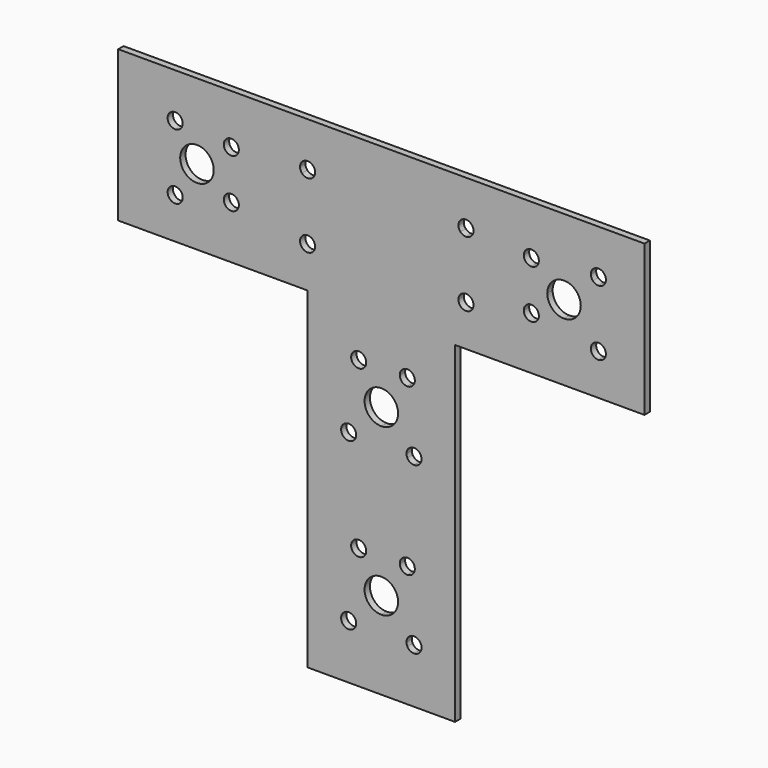
from build123d import *

# Parameters (mm, degrees)
F0_W     = 44
F0_H     = 99
F1_DEPTH = 2
F2_R     = 2.25
F2_R_2   = 5
F3_DEPTH = 2.001


with BuildPart() as f1:
    # F0 (on Front) → F1 (new body)
    with BuildSketch(Plane.XZ):
        Polygon((-78.5, 22.5), (-78.5, -22.5), (-22, -22.5), (22, -22.5), (78.5, -22.5), (78.5, 22.5), align=None)
        with Locations((0, -72)):
            Rectangle(F0_W, F0_H)
    extrude(amount=F1_DEPTH)

    # F2 (on face) → F3 (cut, through all)
    with BuildSketch(Plane.XZ.offset(2)):
        with BuildLine():
            ThreePointArc((7.75, -106.2807764064), (8.5788353904, -107.1711646096), (9.75, -107.5))
            Line((9.75, -107.5), (9.75, -105.25))
            Line((9.75, -105.25), (7.75, -105.25))
            Line((7.75, -105.25), (7.75, -106.2807764064))
        make_face()
        with BuildLine():
            Line((9.75, -105.25), (9.75, -107.5))
            ThreePointArc((9.75, -107.5), (11.3409902577, -106.8409902577), (12, -105.25))
            Line((12, -105.25), (9.75, -105.25))
        make_face()
        with BuildLine():
            Line((9.75, -103), (9.75, -105.25))
            Line((9.75, -105.25), (12, -105.25))
            ThreePointArc((12, -105.25), (11.3409902577, -103.6590097423), (9.75, -103))
        make_face()
        with BuildLine():
            Line((7.75, -105.25), (9.75, -105.25))
            Line((9.75, -105.25), (9.75, -103))
            ThreePointArc((9.75, -103), (8.5788353904, -103.3288353904), (7.75, -104.2192235936))
            Line((7.75, -104.2192235936), (7.75, -105.25))
        make_face()
        with BuildLine():
            ThreePointArc((7.5, -105.25), (7.5633930394, -105.7803300859), (7.75, -106.2807764064))
            Line((7.75, -106.2807764064), (7.75, -105.25))
            Line((7.75, -105.25), (7.5, -105.25))
        make_face()
        with Locations((-9.75, -105.25)):
            Circle(F2_R)
        with Locations((-6.75, -85.25)):
            Circle(F2_R)
        with Locations((-9.75, -55.75)):
            Circle(F2_R)
        with BuildLine():
            ThreePointArc((5, -46), (-3.5355339059, -42.4644660941), (0, -51))
            ThreePointArc((0, -51), (3.5355339059, -49.5355339059), (5, -46))
        make_face()
        with Locations((-6.75, -35.75)):
            Circle(F2_R)
        with BuildLine():
            ThreePointArc((5.5, -35.75), (6.1590097423, -37.3409902577), (7.75, -38))
            Line((7.75, -38), (7.75, -35.75))
            Line((7.75, -35.75), (5.5, -35.75))
        make_face()
        with BuildLine():
            Line((7.75, -35.75), (7.75, -38))
            ThreePointArc((7.75, -38), (9.3409902577, -37.3409902577), (10, -35.75))
            ThreePointArc((10, -35.75), (7.75, -33.5), (5.5, -35.75))
            Line((5.5, -35.75), (7.75, -35.75))
        make_face()
        with Locations((-61.5, -10.25)):
            Circle(F2_R)
        with BuildLine():
            ThreePointArc((-24.25, -10.25), (-22, -12.5), (-19.75, -10.25))
            Line((-19.75, -10.25), (-22, -10.25))
            Line((-22, -10.25), (-24.25, -10.25))
        make_face()
        with BuildLine():
            Line((-22, -10.25), (-19.75, -10.25))
            ThreePointArc((-19.75, -10.25), (-22, -8), (-24.25, -10.25))
            Line((-24.25, -10.25), (-22, -10.25))
        make_face()
        with BuildLine():
            ThreePointArc((27.5, -10.25), (26.8409902577, -8.6590097423), (25.25, -8))
            Line((25.25, -8), (25.25, -10.25))
            Line((25.25, -10.25), (23, -10.25))
            ThreePointArc((23, -10.25), (25.25, -12.5), (27.5, -10.25))
        make_face()
        with BuildLine():
            Line((25.25, -10.25), (25.25, -8))
            ThreePointArc((25.25, -8), (23.6590097423, -8.6590097423), (23, -10.25))
            Line((23, -10.25), (25.25, -10.25))
        make_face()
        with Locations((-44.75, -6.75)):
            Circle(F2_R)
        with Locations((-55, 0)):
            Circle(F2_R_2)
        with Locations((-61.5, 9.25)):
            Circle(F2_R)
        with BuildLine():
            Line((7.5, -105.25), (7.75, -105.25))
            Line((7.75, -105.25), (7.75, -104.2192235936))
            ThreePointArc((7.75, -104.2192235936), (7.5633930394, -104.7196699141), (7.5, -105.25))
        make_face()
        with BuildLine():
            ThreePointArc((0, -90.5), (-5, -95.5), (0, -100.5))
            Line((0, -100.5), (0, -95.5))
            Line((0, -95.5), (0, -90.5))
        make_face()
        with BuildLine():
            Line((0, -95.5), (0, -100.5))
            ThreePointArc((0, -100.5), (3.5355339059, -99.0355339059), (5, -95.5))
            Line((5, -95.5), (0, -95.5))
        make_face()
        with BuildLine():
            Line((9.75, -85.25), (9.75, -86.2807764064))
            ThreePointArc((9.75, -86.2807764064), (9.9366069606, -85.7803300859), (10, -85.25))
            Line((10, -85.25), (9.75, -85.25))
        make_face()
        with BuildLine():
            ThreePointArc((7.75, -87.5), (8.9211646096, -87.1711646096), (9.75, -86.2807764064))
            Line((9.75, -86.2807764064), (9.75, -85.25))
            Line((9.75, -85.25), (7.75, -85.25))
            Line((7.75, -85.25), (7.75, -87.5))
        make_face()
        with BuildLine():
            Line((0, -90.5), (0, -95.5))
            Line((0, -95.5), (5, -95.5))
            ThreePointArc((5, -95.5), (3.5355339059, -91.9644660941), (0, -90.5))
        make_face()
        with BuildLine():
            Line((9.75, -85.25), (10, -85.25))
            ThreePointArc((10, -85.25), (9.9366069606, -84.7196699141), (9.75, -84.2192235936))
            Line((9.75, -84.2192235936), (9.75, -85.25))
        make_face()
        with BuildLine():
            ThreePointArc((5.5, -85.25), (6.1590097423, -86.8409902577), (7.75, -87.5))
            Line((7.75, -87.5), (7.75, -85.25))
            Line((7.75, -85.25), (5.5, -85.25))
        make_face()
        with BuildLine():
            Line((7.75, -85.25), (9.75, -85.25))
            Line((9.75, -85.25), (9.75, -84.2192235936))
            ThreePointArc((9.75, -84.2192235936), (8.9211646096, -83.3288353904), (7.75, -83))
            Line((7.75, -83), (7.75, -85.25))
        make_face()
        with BuildLine():
            Line((5.5, -85.25), (7.75, -85.25))
            Line((7.75, -85.25), (7.75, -83))
            ThreePointArc((7.75, -83), (6.1590097423, -83.6590097423), (5.5, -85.25))
        make_face()
        with BuildLine():
            ThreePointArc((7.75, -56.7807764064), (8.5788353904, -57.6711646096), (9.75, -58))
            Line((9.75, -58), (9.75, -55.75))
            Line((9.75, -55.75), (7.75, -55.75))
            Line((7.75, -55.75), (7.75, -56.7807764064))
        make_face()
        with BuildLine():
            Line((9.75, -55.75), (9.75, -58))
            ThreePointArc((9.75, -58), (11.3409902577, -57.3409902577), (12, -55.75))
            ThreePointArc((12, -55.75), (10.2803300859, -53.5633930394), (7.75, -54.7192235936))
            Line((7.75, -54.7192235936), (7.75, -55.75))
            Line((7.75, -55.75), (9.75, -55.75))
        make_face()
        with BuildLine():
            ThreePointArc((49.5, 0), (50.9644660941, -3.5355339059), (54.5, -5))
            Line((54.5, -5), (54.5, 0))
            Line((54.5, 0), (49.5, 0))
        make_face()
        with BuildLine():
            Line((54.5, 0), (54.5, -5))
            ThreePointArc((54.5, -5), (58.0355339059, -3.5355339059), (59.5, 0))
            Line((59.5, 0), (54.5, 0))
        make_face()
        with BuildLine():
            Line((7.75, -55.75), (7.5, -55.75))
            ThreePointArc((7.5, -55.75), (7.5633930394, -56.2803300859), (7.75, -56.7807764064))
            Line((7.75, -56.7807764064), (7.75, -55.75))
        make_face()
        with BuildLine():
            ThreePointArc((7.75, -54.7192235936), (7.5633930394, -55.2196699141), (7.5, -55.75))
            Line((7.5, -55.75), (7.75, -55.75))
            Line((7.75, -55.75), (7.75, -54.7192235936))
        make_face()
        with BuildLine():
            Line((44.75, 9.25), (44.75, 10))
            ThreePointArc((44.75, 10), (43.8314413465, 9.8039595906), (43.0729490169, 9.25))
            Line((43.0729490169, 9.25), (44.75, 9.25))
        make_face()
        with BuildLine():
            ThreePointArc((46.4270509831, 9.25), (45.6685586535, 9.8039595906), (44.75, 10))
            Line((44.75, 10), (44.75, 9.25))
            Line((44.75, 9.25), (46.4270509831, 9.25))
        make_face()
        with BuildLine():
            Line((49.5, 0), (54.5, 0))
            Line((54.5, 0), (59.5, 0))
            ThreePointArc((59.5, 0), (54.5, 5), (49.5, 0))
        make_face()
        with BuildLine():
            ThreePointArc((64.75, -8), (62.5, -10.25), (64.75, -12.5))
            Line((64.75, -12.5), (64.75, -10.25))
            Line((64.75, -10.25), (64.75, -8))
        make_face()
        with BuildLine():
            Line((64.75, -10.25), (64.75, -12.5))
            ThreePointArc((64.75, -12.5), (66.3409902577, -11.8409902577), (67, -10.25))
            Line((67, -10.25), (64.75, -10.25))
        make_face()
        with BuildLine():
            ThreePointArc((47, 7.75), (46.8518878077, 8.552849702), (46.4270509831, 9.25))
            Line((46.4270509831, 9.25), (44.75, 9.25))
            Line((44.75, 9.25), (44.75, 7.75))
            Line((44.75, 7.75), (47, 7.75))
        make_face()
        with BuildLine():
            Line((44.75, 9.25), (43.0729490169, 9.25))
            ThreePointArc((43.0729490169, 9.25), (42.6481121923, 8.552849702), (42.5, 7.75))
            Line((42.5, 7.75), (44.75, 7.75))
            Line((44.75, 7.75), (44.75, 9.25))
        make_face()
        with BuildLine():
            Line((64.75, -8), (64.75, -10.25))
            Line((64.75, -10.25), (67, -10.25))
            ThreePointArc((67, -10.25), (66.3409902577, -8.6590097423), (64.75, -8))
        make_face()
        with BuildLine():
            ThreePointArc((44.75, 5.5), (46.3409902577, 6.1590097423), (47, 7.75))
            Line((47, 7.75), (44.75, 7.75))
            Line((44.75, 7.75), (44.75, 5.5))
        make_face()
        with BuildLine():
            Line((64.75, 9.25), (62.5, 9.25))
            ThreePointArc((62.5, 9.25), (62.6481121923, 8.447150298), (63.0729490169, 7.75))
            Line((63.0729490169, 7.75), (64.75, 7.75))
            Line((64.75, 7.75), (64.75, 9.25))
        make_face()
        with BuildLine():
            ThreePointArc((67, 9.25), (64.75, 11.5), (62.5, 9.25))
            Line((62.5, 9.25), (64.75, 9.25))
            Line((64.75, 9.25), (64.75, 7.75))
            Line((64.75, 7.75), (66.4270509831, 7.75))
            ThreePointArc((66.4270509831, 7.75), (66.8518878077, 8.447150298), (67, 9.25))
        make_face()
        with BuildLine():
            Line((44.75, 7.75), (42.5, 7.75))
            ThreePointArc((42.5, 7.75), (43.1590097423, 6.1590097423), (44.75, 5.5))
            Line((44.75, 5.5), (44.75, 7.75))
        make_face()
        with BuildLine():
            ThreePointArc((26.9270509831, 7.75), (27.3518878077, 8.447150298), (27.5, 9.25))
            Line((27.5, 9.25), (25.25, 9.25))
            Line((25.25, 9.25), (25.25, 7.75))
            Line((25.25, 7.75), (26.9270509831, 7.75))
        make_face()
        with BuildLine():
            Line((25.25, 9.25), (27.5, 9.25))
            ThreePointArc((27.5, 9.25), (25.25, 11.5), (23, 9.25))
            Line((23, 9.25), (25.25, 9.25))
        make_face()
        with BuildLine():
            ThreePointArc((64.75, 7), (65.6685586535, 7.1960404094), (66.4270509831, 7.75))
            Line((66.4270509831, 7.75), (64.75, 7.75))
            Line((64.75, 7.75), (64.75, 7))
        make_face()
        with BuildLine():
            ThreePointArc((47, -6.75), (46.3409902577, -5.1590097423), (44.75, -4.5))
            Line((44.75, -4.5), (44.75, -6.75))
            Line((44.75, -6.75), (42.5, -6.75))
            ThreePointArc((42.5, -6.75), (44.75, -9), (47, -6.75))
        make_face()
        with BuildLine():
            Line((44.75, -6.75), (44.75, -4.5))
            ThreePointArc((44.75, -4.5), (43.1590097423, -5.1590097423), (42.5, -6.75))
            Line((42.5, -6.75), (44.75, -6.75))
        make_face()
        with BuildLine():
            ThreePointArc((63.0729490169, 7.75), (63.8314413465, 7.1960404094), (64.75, 7))
            Line((64.75, 7), (64.75, 7.75))
            Line((64.75, 7.75), (63.0729490169, 7.75))
        make_face()
        with BuildLine():
            ThreePointArc((25.25, 7), (26.1685586535, 7.1960404094), (26.9270509831, 7.75))
            Line((26.9270509831, 7.75), (25.25, 7.75))
            Line((25.25, 7.75), (25.25, 7))
        make_face()
        with BuildLine():
            Line((25.25, 7.75), (25.25, 9.25))
            Line((25.25, 9.25), (23, 9.25))
            ThreePointArc((23, 9.25), (23.1481121923, 8.447150298), (23.5729490169, 7.75))
            Line((23.5729490169, 7.75), (25.25, 7.75))
        make_face()
        with BuildLine():
            ThreePointArc((23.5729490169, 7.75), (24.3314413465, 7.1960404094), (25.25, 7))
            Line((25.25, 7), (25.25, 7.75))
            Line((25.25, 7.75), (23.5729490169, 7.75))
        make_face()
        with BuildLine():
            ThreePointArc((-20.3229490169, 7.75), (-19.8981121923, 8.447150298), (-19.75, 9.25))
            Line((-19.75, 9.25), (-22, 9.25))
            Line((-22, 9.25), (-24.25, 9.25))
            ThreePointArc((-24.25, 9.25), (-24.1018878077, 8.447150298), (-23.6770509831, 7.75))
            Line((-23.6770509831, 7.75), (-20.3229490169, 7.75))
        make_face()
        with BuildLine():
            Line((-22, 9.25), (-19.75, 9.25))
            ThreePointArc((-19.75, 9.25), (-22, 11.5), (-24.25, 9.25))
            Line((-24.25, 9.25), (-22, 9.25))
        make_face()
        with BuildLine():
            ThreePointArc((-23.6770509831, 7.75), (-22, 7), (-20.3229490169, 7.75))
            Line((-20.3229490169, 7.75), (-23.6770509831, 7.75))
        make_face()
        with BuildLine():
            ThreePointArc((-42.5, 7.75), (-42.6481121923, 8.552849702), (-43.0729490169, 9.25))
            Line((-43.0729490169, 9.25), (-46.4270509831, 9.25))
            ThreePointArc((-46.4270509831, 9.25), (-45.552849702, 5.6481121923), (-42.5, 7.75))
        make_face()
        with BuildLine():
            Line((-46.4270509831, 9.25), (-43.0729490169, 9.25))
            ThreePointArc((-43.0729490169, 9.25), (-44.75, 10), (-46.4270509831, 9.25))
        make_face()
    extrude(amount=-F3_DEPTH, mode=Mode.SUBTRACT)


solid = f1.part
